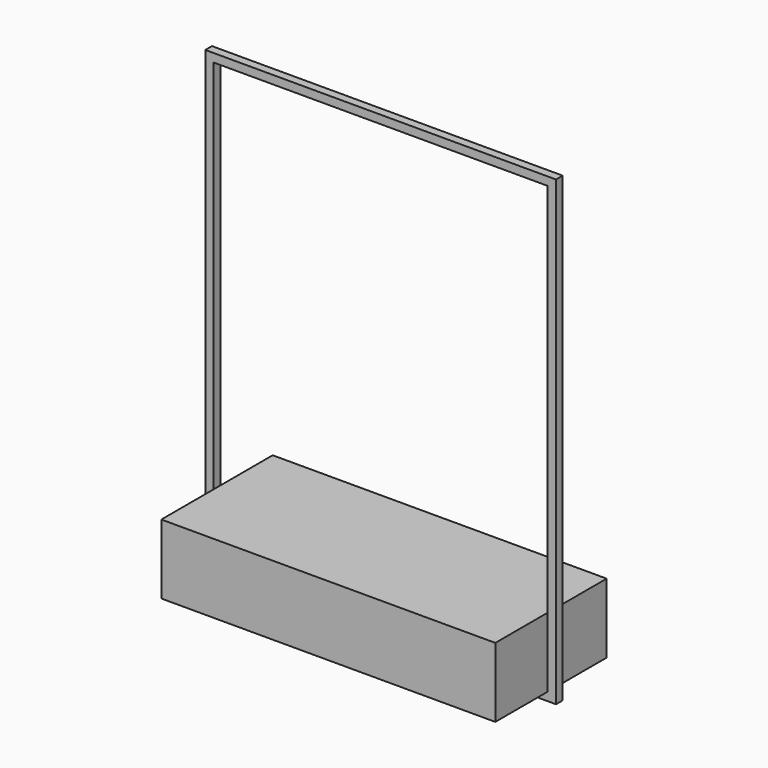
from build123d import *

# Parameters (mm, degrees)
F0_W     = 1200
F0_H     = 500
F1_DEPTH = 250
F2_W     = 1260
F2_H     = 1660
F2_W_2   = 1200
F2_H_2   = 1600
F3_DEPTH = 15
F4_W     = 1000
F4_H     = 300
F4_W_2   = 940
F4_H_2   = 240
F5_DEPTH = 30


with BuildPart() as f1:
    # F0 (on Top) → F1 (new body)
    with BuildSketch(Plane.XY):
        Rectangle(F0_W, F0_H)
    extrude(amount=F1_DEPTH)


with BuildPart() as f3:
    # F2 (on Front) → F3 (new body, symmetric)
    with BuildSketch(Plane.XZ):
        with Locations((0, 800)):
            Rectangle(F2_W, F2_H)
        with Locations((0, 800)):
            Rectangle(F2_W_2, F2_H_2, mode=Mode.SUBTRACT)
    extrude(amount=F3_DEPTH, both=True)

    # F4 (on face) → F5 (join)
    with BuildSketch(Plane(origin=(0, 0, 0), x_dir=(1, 0, 0), z_dir=(0, 0, -1))):
        Rectangle(F4_W, F4_H)
        Rectangle(F4_W_2, F4_H_2, mode=Mode.SUBTRACT)
    extrude(amount=F5_DEPTH)


solid = Compound([f1.part, f3.part])
